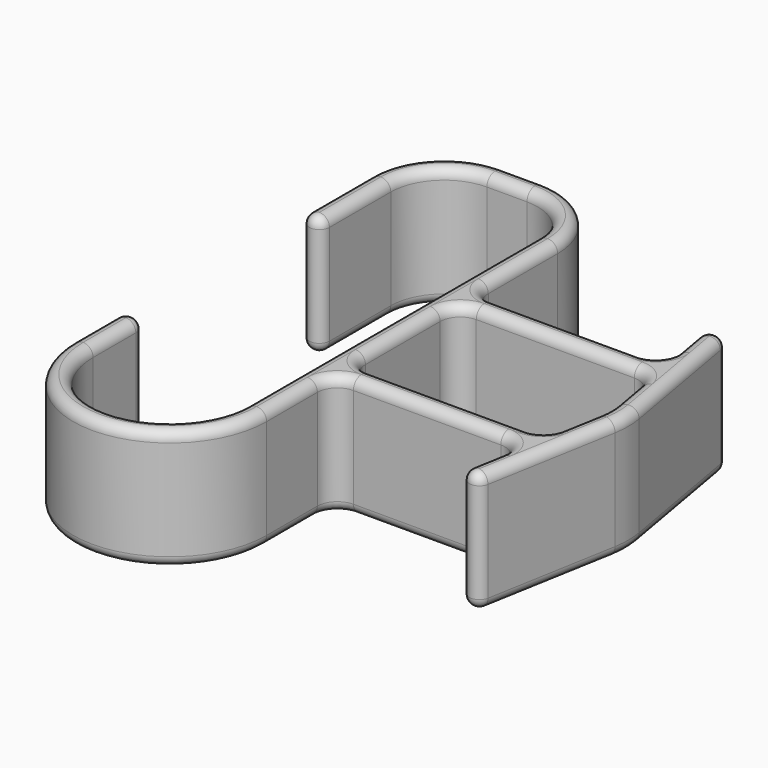
from build123d import *

# Parameters (mm, degrees)
F1_DEPTH = 18
F2_R     = 1.49999


# Not quite as in the source:
# - a fillet or chamfer is up to 0.001 mm smaller than in the source, because OpenCascade refuses the exact size


with BuildPart() as f1:
    # F0 (on Top) → F1 (new body)
    with BuildSketch(Plane.XY):
        with BuildLine():
            ThreePointArc((4, 29), (6.3431457505, 34.6568542495), (12, 37))
            Line((12, 37), (18, 37))
            ThreePointArc((18, 37), (23.6568542495, 34.6568542495), (26, 29))
            Line((26, 29), (26, -25.5))
            ThreePointArc((26, -25.5), (14.5, -37), (3, -25.5))
            Line((3, -25.5), (3, -17.5))
            ThreePointArc((3, -17.5), (1.5, -16), (0, -17.5))
            Line((0, -17.5), (0, -25.5))
            ThreePointArc((0, -25.5), (14.5, -40), (29, -25.5))
            Line((29, -25.5), (29, -16))
            ThreePointArc((29, -16), (29.8786796564, -13.8786796564), (32, -13))
            Line((32, -13), (54.0862086374, -13))
            ThreePointArc((54.0862086374, -13), (56.3843419667, -14.0716371709), (57.0406318964, -16.520944533))
            Line((57.0406318964, -16.520944533), (56.2086183674, -21.2395277335))
            ThreePointArc((56.2086183674, -21.2395277335), (57.4253577304, -22.9772116295), (59.1630416265, -21.7604722665))
            Line((59.1630416265, -21.7604722665), (62.6019548346, -2.2574263097))
            ThreePointArc((62.6019548346, -2.2574263097), (62.7994540455, 0), (62.6019548346, 2.2574263097))
            Line((62.6019548346, 2.2574263097), (59.1630416265, 21.7604722665))
            ThreePointArc((59.1630416265, 21.7604722665), (57.4253577304, 22.9772116295), (56.2086183674, 21.2395277335))
            Line((56.2086183674, 21.2395277335), (57.0406318964, 16.520944533))
            ThreePointArc((57.0406318964, 16.520944533), (56.3843419667, 14.0716371709), (54.0862086374, 13))
            Line((54.0862086374, 13), (32, 13))
            ThreePointArc((32, 13), (29.8786796564, 13.8786796564), (29, 16))
            Line((29, 16), (29, 29))
            ThreePointArc((29, 29), (25.7781745931, 36.7781745931), (18, 40))
            Line((18, 40), (12, 40))
            ThreePointArc((12, 40), (4.2218254069, 36.7781745931), (1, 29))
            Line((1, 29), (1, 17.5))
            ThreePointArc((1, 17.5), (2.5, 16), (4, 17.5))
            Line((4, 17.5), (4, 29))
        make_face()
        with BuildLine():
            ThreePointArc((29, 6.9999995083), (29.8786796564, 9.1213198518), (32, 9.9999995083))
            Line((32, 9.9999995083), (55.6731515504, 9.9999995083))
            ThreePointArc((55.6731515504, 9.9999995083), (57.6015143795, 9.2981328376), (58.6275748095, 7.5209440413))
            Line((58.6275748095, 7.5209440413), (59.6475315756, 1.7364817767))
            ThreePointArc((59.6475315756, 1.7364817767), (59.7994540455, 0), (59.6475315756, -1.7364817767))
            Line((59.6475315756, -1.7364817767), (58.6275748095, -7.5209440413))
            ThreePointArc((58.6275748095, -7.5209440413), (57.6015143795, -9.2981328376), (55.6731515504, -9.9999995083))
            Line((55.6731515504, -9.9999995083), (32, -9.9999995083))
            ThreePointArc((32, -9.9999995083), (29.8786796564, -9.1213198518), (29, -6.9999995083))
            Line((29, -6.9999995083), (29, 6.9999995083))
        make_face(mode=Mode.SUBTRACT)
    extrude(amount=F1_DEPTH)

    # F2 (radius 1.5 in the source; OpenCascade refuses exactly that, so slightly less here)
    f2_edges = [f1.edges().sort_by_distance(p)[0] for p in [
        (4, 23.25, 18),
        (29.87868, 9.12132, 18),
        (23.656854, 34.656854, 0),
        (43.836576, 10, 0),
    ]]
    fillet(f2_edges, radius=F2_R)


solid = f1.part
